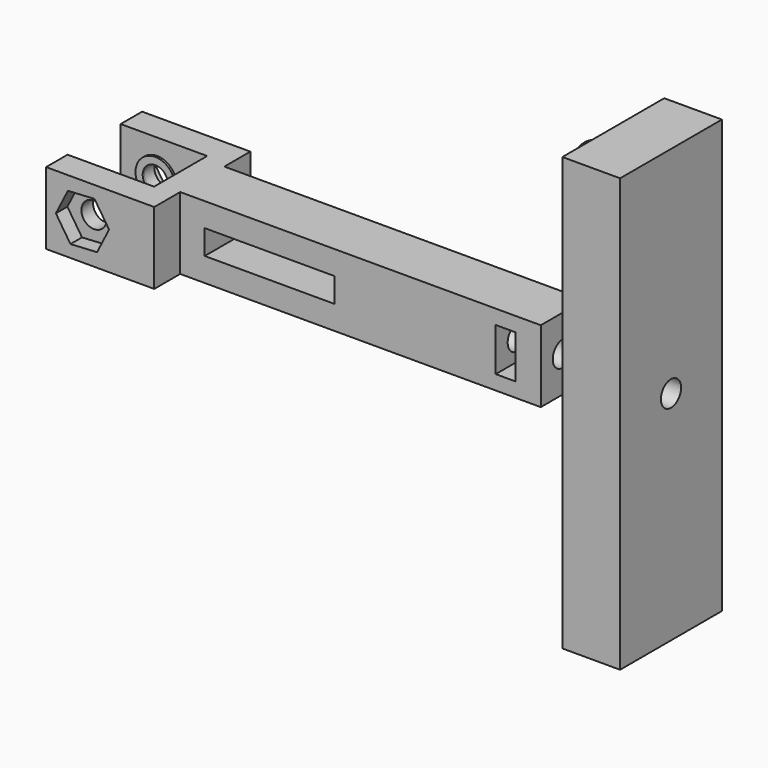
from build123d import *

# Parameters (mm, degrees)
F0_W      = 50
F0_H      = 3.825
F1_DEPTH  = 10
F2_R      = 1.75
F3_DEPTH  = 16.651
F4_W      = 18
F4_H      = 3.4
F4_W_2    = 2.75
F4_H_2    = 6
F5_DEPTH  = 12.151
F6_R      = 1.75
F7_DEPTH  = 15
F10_DEPTH = 2
F11_W     = 17.65
F11_H     = 60
F12_DEPTH = 8
F13_R     = 1.75
F14_DEPTH = 80.001
F15_R     = 2.75
F15_R_2   = 1.75
F16_DEPTH = 0.3
F17_R     = 1.75
F18_DEPTH = 2
F19_R     = 3.75
F20_DEPTH = 4


# Not quite as in the source:
# - a pattern or mirror of a feature is missing from the dataset's text; its kind, count and spacing are read off the source's solid


with BuildPart() as f1:
    # F0 (on Top) → F1 (new body)
    with BuildSketch(Plane.XY):
        Polygon((0, -3.825), (0, 0), (-3, 0), (-3, -4.6), (-15, -4.6), (-15, -8.325), (0, -8.325), align=None)
        Polygon((-3, 0), (0, 0), (0, 3.825), (0, 8.325), (-15, 8.325), (-15, 4.6), (-3, 4.6), align=None)
        with Locations((25, 1.9125)):
            Rectangle(F0_W, F0_H)
        with Locations((25, -1.9125)):
            Rectangle(F0_W, F0_H)
    extrude(amount=F1_DEPTH)

    # F2 (on face) → F3 (cut, through all)
    with BuildSketch(Plane.XZ.offset(8.325)):
        with Locations((-9.9527407438, 5)):
            Circle(F2_R)
    extrude(amount=-F3_DEPTH, mode=Mode.SUBTRACT)

    # F4 (on face) → F5 (cut, through all)
    with BuildSketch(Plane.XZ.offset(3.825)):
        with Locations((12.4002694301, 5)):
            Rectangle(F4_W, F4_H)
        with Locations((45.125, 5)):
            Rectangle(F4_W_2, F4_H_2)
    extrude(amount=-F5_DEPTH, mode=Mode.SUBTRACT)

    # F6 (on face) → F7 (cut)
    with BuildSketch(Plane.YZ.offset(50)):
        with Locations((0, 5)):
            Circle(F6_R)
    extrude(amount=-F7_DEPTH, mode=Mode.SUBTRACT)

    # F15 (on face) → F16 (join)
    with BuildSketch(Plane.XZ.offset(-4.6)):
        with Locations((-9.9527407438, 5)):
            Circle(F15_R)
        with Locations((-9.9527407438, 5)):
            Circle(F15_R_2, mode=Mode.SUBTRACT)
    f16 = extrude(amount=F16_DEPTH)

    # F16_copies: F16 across plane
    add(f16.mirror(Plane(origin=(0, 0, 0), x_dir=(0, 0, -1), z_dir=(0, -1, 0))))

    # F17 (on face) → F18 (cut)
    with BuildSketch(Plane.XZ.offset(8.325)):
        Polygon((-7.9284293953, 1.9088033227), (-6.2635302189, 5.2075067143), (-8.2878415673, 8.2987033916), (-11.9770520922, 8.0911966773), (-13.6419512686, 4.7924932857), (-11.6176399202, 1.7012966084), align=None)
        with Locations((-9.9527407438, 5)):
            Circle(F17_R, mode=Mode.SUBTRACT)
    f18 = extrude(amount=-F18_DEPTH, mode=Mode.SUBTRACT)

    # F18_copies: F18 across plane
    add(f18.mirror(Plane.ZX), mode=Mode.SUBTRACT)


with BuildPart() as f10:
    # F9 (on offset) → F10 (new body)
    with BuildSketch(Plane.YZ.offset(55)):
        Polygon((3.825, 0), (3.825, 10), (3.825, 19.8484882712), (-3.825, 19.8484882712), (-3.825, 10), (-3.825, 0), (-3.825, -10.1515117288), (3.825, -10.1515117288), align=None)
    extrude(amount=F10_DEPTH)

    # F11 (on face) → F12 (join)
    with BuildSketch(Plane.YZ.offset(57)):
        with Locations((0, 4.8484882712)):
            Rectangle(F11_W, F11_H)
    extrude(amount=F12_DEPTH)

    # F13 (on face) → F14 (cut, through all)
    with BuildSketch(Plane.YZ.offset(65)):
        with Locations((0, 5)):
            Circle(F13_R)
    extrude(amount=-F14_DEPTH, mode=Mode.SUBTRACT)

    # F19 (on face) → F20 (join)
    with BuildSketch(Plane(origin=(57, 0, 0), x_dir=(0, -1, 0), z_dir=(-1, 0, 0))):
        with Locations((0, 28)):
            Circle(F19_R)
        with Locations((0, -18)):
            Circle(F19_R)
    extrude(amount=F20_DEPTH)


solid = Compound([f1.part, f10.part])
